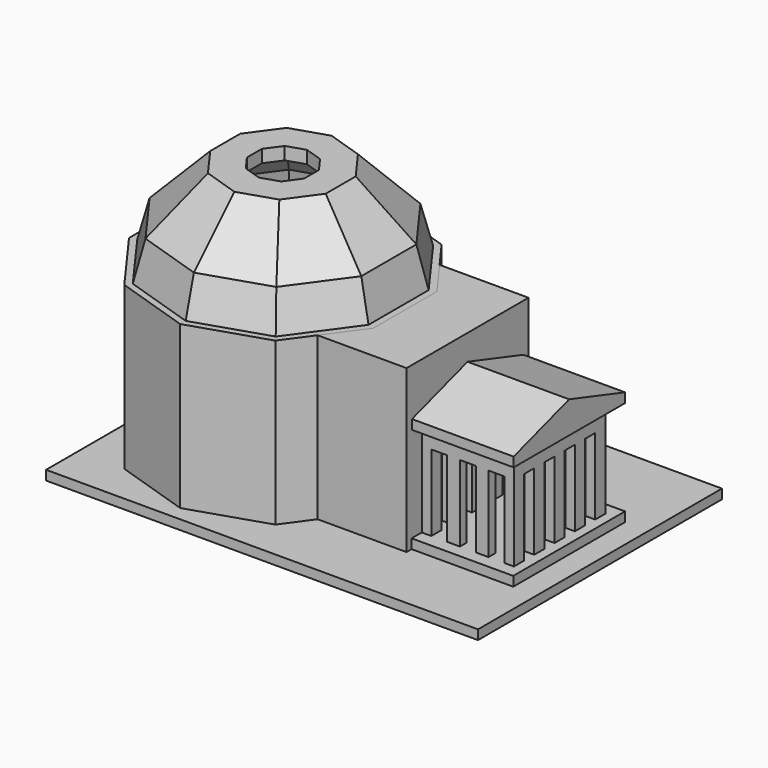
from build123d import *

# Parameters (mm, degrees)
F0_W      = 215.9
F0_H      = 152.4
F1_DEPTH  = 4.7625
F3_DEPTH  = 80.9625
F4_T      = -4.7625
F6_DEPTH  = 25.4
F7_DEPTH  = 80.9625
F8_W      = 50.8
F8_H      = 69.85
F9_DEPTH  = 4.7625
F10_W     = 4.7625
F10_H     = 6.35
F10_W_2   = 6.35
F10_H_2   = 4.2333333333
F11_DEPTH = 38.1
F12_W     = 46.0375
F12_H     = 57.15
F12_W_2   = 36.5125
F12_H_2   = 47.625
F13_DEPTH = 9.525
F15_DEPTH = 50.8


with BuildPart() as f1:
    # F0 (on Top) → F1 (new body)
    with BuildSketch(Plane.XY):
        with Locations((-0.2590711229, 4.5428941069)):
            Rectangle(F0_W, F0_H)
    extrude(amount=F1_DEPTH)


with BuildPart() as f3:
    # F2 (on face) → F3 (new body)
    with BuildSketch(Plane.XY.offset(4.7625)):
        Polygon((-9.3912329416, 51.9516119643), (-47.136288432, 64.2157239285), (-84.8813439225, 51.9516119643), (-108.2090711229, 19.84375), (-108.2090711229, -19.84375), (-84.8813439225, -51.9516119643), (-47.136288432, -64.2157239285), (-9.3912329416, -51.9516119643), (0.6725522319, -38.1), (13.9364942588, -19.84375), (13.9364942588, 19.84375), (0.6725522319, 38.1), align=None)
    extrude(amount=F3_DEPTH)

    # F4
    f4_openings = [f3.faces().sort_by_distance(p)[0] for p in [
        (-47.136288, 0, 4.7625),
    ]]
    offset(amount=F4_T, openings=f4_openings)

    # F5 (on face) → F6 (cut)
    with BuildSketch(Plane.XY.offset(85.725)):
        Polygon((-73.1077964368, 35.7467140651), (-89.1590711229, 13.6540297868), (-89.1590711229, -13.6540297868), (-73.1077964368, -35.7467140651), (-47.136288432, -44.1853685568), (-21.1647804273, -35.7467140651), (-5.1135057412, -13.6540297868), (-5.1135057412, 13.6540297868), (-21.1647804273, 35.7467140651), (-47.136288432, 44.1853685568), align=None)
    extrude(amount=-F6_DEPTH, mode=Mode.SUBTRACT)


with BuildPart() as f7:
    # F2 (on face) → F7 (new body, through all)
    with BuildSketch(Plane.XY.offset(4.7625)):
        Polygon((45.1225522319, 38.1), (0.6725522319, 38.1), (13.9364942588, 19.84375), (13.9364942588, -19.84375), (0.6725522319, -38.1), (45.1225522319, -38.1), (45.1225522319, 0), align=None)
    extrude(amount=F7_DEPTH)


with BuildPart() as f9:
    # F8 (on face) → F9 (new body)
    with BuildSketch(Plane.XY.offset(4.7625)):
        with Locations((70.5225522319, 0)):
            Rectangle(F8_W, F8_H)
    extrude(amount=F9_DEPTH)

    # F10 (on face) → F11 (join)
    with BuildSketch(Plane.XY.offset(9.525)):
        with Locations((88.7788022319, 25.4)):
            Rectangle(F10_W, F10_H)
        with Locations((88.7788022319, 12.7)):
            Rectangle(F10_W, F10_H)
        with Locations((88.7788022319, 0)):
            Rectangle(F10_W, F10_H)
        with Locations((88.7788022319, -12.7)):
            Rectangle(F10_W, F10_H)
        with Locations((88.7788022319, -25.4)):
            Rectangle(F10_W, F10_H)
        with Locations((75.2850522319, 26.4583333333)):
            Rectangle(F10_W_2, F10_H_2)
        with Locations((47.5038022319, 25.4)):
            Rectangle(F10_W, F10_H)
        with Locations((47.5038022319, 12.7)):
            Rectangle(F10_W, F10_H)
        with Locations((47.5038022319, 0)):
            Rectangle(F10_W, F10_H)
        with Locations((47.5038022319, -12.7)):
            Rectangle(F10_W, F10_H)
        with Locations((47.5038022319, -25.4)):
            Rectangle(F10_W, F10_H)
        with Locations((75.2850522319, -26.4583333333)):
            Rectangle(F10_W_2, F10_H_2)
        with Locations((60.9975522319, -26.4583333333)):
            Rectangle(F10_W_2, F10_H_2)
        with Locations((60.9975522319, 26.4583333333)):
            Rectangle(F10_W_2, F10_H_2)
    extrude(amount=F11_DEPTH)

    # F12 (on face) → F13 (join)
    with BuildSketch(Plane.XY.offset(47.625)):
        with Locations((68.1413022319, 0)):
            Rectangle(F12_W, F12_H)
        with Locations((68.1413022319, 0)):
            Rectangle(F12_W_2, F12_H_2, mode=Mode.SUBTRACT)
    extrude(amount=F13_DEPTH)

    # F14 (on face) → F15 (join)
    with BuildSketch(Plane.YZ.offset(95.9225522319)):
        Polygon((-34.6816889942, 57.15), (-28.3316889942, 57.15), (28.575, 57.15), (34.925, 57.15), (34.925, 61.9125), (0, 73.025), (-34.6816889942, 61.9125), align=None)
    extrude(amount=-F15_DEPTH)


with BuildPart() as f18:
    # F18: sweep along a path in F5
    with BuildLine(Plane.XY.offset(85.725)) as f18_path:
        Line((-5.1135057412, -13.6540297868), (-21.1647804273, -35.7467140651))
        Line((-21.1647804273, -35.7467140651), (-47.136288432, -44.1853685568))
        Line((-47.136288432, -44.1853685568), (-73.1077964368, -35.7467140651))
        Line((-73.1077964368, -35.7467140651), (-89.1590711229, -13.6540297868))
        Line((-89.1590711229, -13.6540297868), (-89.1590711229, 13.6540297868))
        Line((-89.1590711229, 13.6540297868), (-73.1077964368, 35.7467140651))
        Line((-73.1077964368, 35.7467140651), (-47.136288432, 44.1853685568))
        Line((-47.136288432, 44.1853685568), (-21.1647804273, 35.7467140651))
        Line((-21.1647804273, 35.7467140651), (-5.1135057412, 13.6540297868))
        Line((-5.1135057412, 13.6540297868), (-5.1135057412, -13.6540297868))
    # F17 (on mid) → F18 (sweep)
    with BuildSketch(Plane(origin=(-4.5011150194, -13.8530075941, 0), x_dir=(0.9510565163, -0.3090169944, 0), z_dir=(-0.3090169944, -0.9510565163, 0))):
        Polygon((5.1206323029, 101.6), (9.3743257327, 85.725), (15.9483294784, 85.725), (10.8138865512, 104.8870018728), (-14.474111576, 130.175), (-29.8043676971, 130.175), (-29.8043676971, 123.825), (-17.1043676971, 123.825), align=None)
    sweep(path=f18_path.line, transition=Transition.RIGHT)


solid = Compound([f1.part, f3.part, f7.part, f9.part, f18.part])
